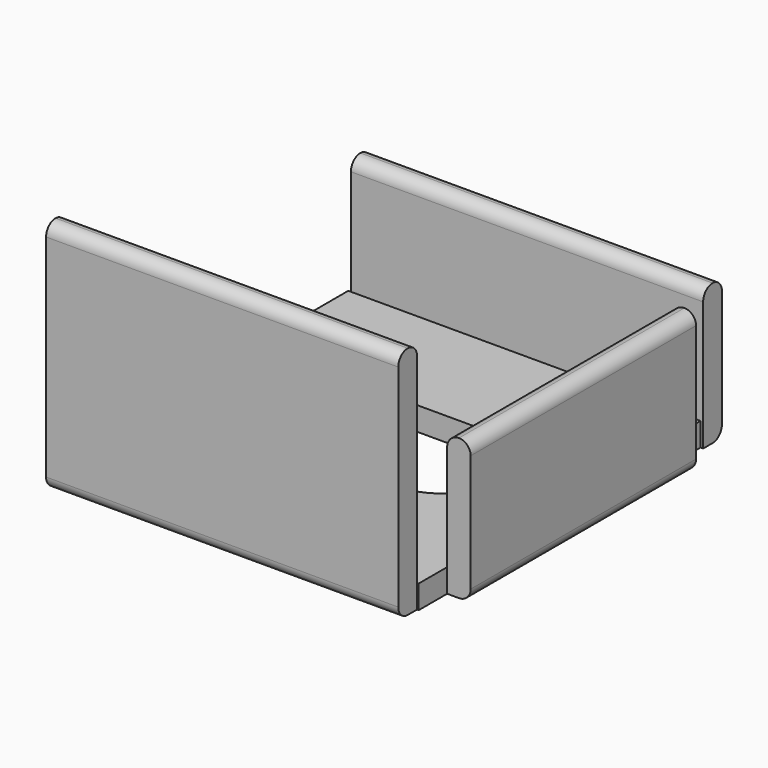
from build123d import *

# Parameters (mm, degrees)
F9_W      = 12
F9_H      = 6
F10_DEPTH = 1
F8_W      = 15
F8_H      = 6
F11_DEPTH = 1
F7_W      = 15
F7_H      = 10
F12_DEPTH = 1
F0_W      = 15
F0_H      = 15
F13_DEPTH = 1
F14_R     = 0.5
F15_R     = 0.49999
F15_2_R   = 0.49999
F16_R     = 0.49999
F16_2_R   = 0.49999
F17_DEPTH = 1


# Not quite as in the source:
# - a fillet or chamfer is up to 0.001 mm smaller than in the source, because OpenCascade refuses the exact size


with BuildPart() as f10:
    # F9 (on plane+point) → F10 (new body)
    with BuildSketch(Plane.YZ.offset(7.5)):
        with Locations((0.0150063767, 3)):
            Rectangle(F9_W, F9_H)
    extrude(amount=F10_DEPTH)

    # F14
    f14_edges = [f10.edges().sort_by_distance(p)[0] for p in [
        (8.5, 0.015006, 6),
    ]]
    fillet(f14_edges, radius=F14_R)

    # F15 (radius 0.5 in the source; OpenCascade refuses exactly that, so slightly less here)
    f15_edges = [f10.edges().sort_by_distance(p)[0] for p in [
        (7.5, 0.015006, 6),
        (8.5, 0.015006, 0),
    ]]
    fillet(f15_edges, radius=F15_R)

    # F0 (on Top) → F17 (cut)
    with BuildSketch(Plane.XY):
        with BuildLine():
            Line((2.5, 2.5), (-2.5, 2.5))
            ThreePointArc((-2.5, 2.5), (-4.267766953, 1.767766953), (-5, 0))
            ThreePointArc((-5, 0), (-4.267766953, -1.767766953), (-2.5, -2.5))
            Line((-2.5, -2.5), (2.5, -2.5))
            ThreePointArc((2.5, -2.5), (4.267766953, -1.767766953), (5, 0))
            ThreePointArc((5, 0), (4.267766953, 1.767766953), (2.5, 2.5))
        make_face()
    extrude(amount=F17_DEPTH, mode=Mode.SUBTRACT)


with BuildPart() as f11:
    # F8 (on plane+point) → F11 (new body)
    with BuildSketch(Plane.XZ.offset(-7.5)):
        with Locations((0.1134890686, 3)):
            Rectangle(F8_W, F8_H)
    extrude(amount=-F11_DEPTH)

    # F0 (on Top) → F13 (join)
    with BuildSketch(Plane.XY):
        Rectangle(F0_W, F0_H)
        with BuildLine():
            ThreePointArc((-5, 0), (-4.267766953, 1.767766953), (-2.5, 2.5))
            Line((-2.5, 2.5), (2.5, 2.5))
            ThreePointArc((2.5, 2.5), (4.267766953, 1.767766953), (5, 0))
            ThreePointArc((5, 0), (4.267766953, -1.767766953), (2.5, -2.5))
            Line((2.5, -2.5), (-2.5, -2.5))
            ThreePointArc((-2.5, -2.5), (-4.267766953, -1.767766953), (-5, 0))
        make_face(mode=Mode.SUBTRACT)
    extrude(amount=F13_DEPTH)

    # F16#2 (radius 0.5 in the source; OpenCascade refuses exactly that, so slightly less here)
    f16_2_edges = [f11.edges().sort_by_distance(p)[0] for p in [
        (0.113489, 8.5, 0),
        (0.113489, 8.5, 6),
        (0.113489, 7.5, 6),
    ]]
    fillet(f16_2_edges, radius=F16_2_R)


with BuildPart() as f12:
    # F7 (on plane+point) → F12 (new body)
    with BuildSketch(Plane.XZ.offset(7.5)):
        with Locations((-0.0702422911, 5)):
            Rectangle(F7_W, F7_H)
    extrude(amount=F12_DEPTH)

    # F15#2 (radius 0.5 in the source; OpenCascade refuses exactly that, so slightly less here)
    f15_2_edges = [f12.edges().sort_by_distance(p)[0] for p in [
        (-0.070242, -8.5, 10),
        (-0.070242, -7.5, 10),
    ]]
    fillet(f15_2_edges, radius=F15_2_R)

    # F16 (radius 0.5 in the source; OpenCascade refuses exactly that, so slightly less here)
    f16_edges = [f12.edges().sort_by_distance(p)[0] for p in [
        (-0.070242, -8.5, 0),
    ]]
    fillet(f16_edges, radius=F16_R)


solid = Compound([f10.part, f11.part, f12.part])
